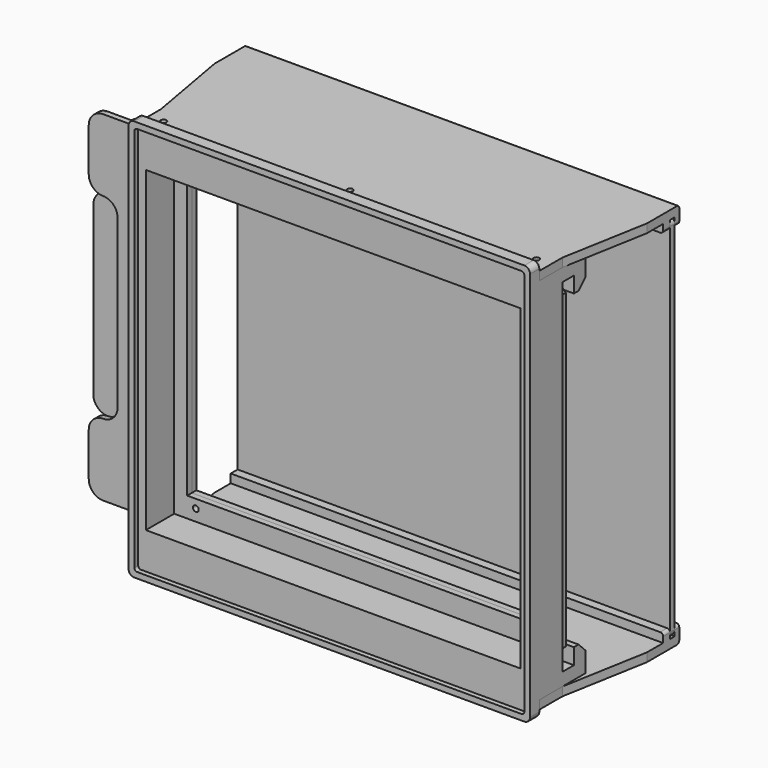
from build123d import *

# Parameters (mm, degrees)
F0_W      = 139.3
F0_H      = 139.3
F0_W_2    = 130
F0_H_2    = 110
F1_DEPTH  = 2.3
F2_W      = 139.3
F2_H      = 128
F2_W_2    = 130
F2_H_2    = 110
F3_DEPTH  = 10
F4_W      = 139.3
F4_H      = 139.3
F4_W_2    = 135.3
F4_H_2    = 135.3
F5_DEPTH  = 1.7
F6_R      = 1
F7_R      = 2
F8_W      = 162.3
F8_H      = 118
F8_W_2    = 121
F8_H_2    = 96
F9_DEPTH  = 2
F10_R     = 1
F11_DEPTH = 25
F12_SIZE  = 5
F13_R     = 1
F13_W     = 121
F13_H     = 96
F14_DEPTH = 2
F15_W     = 10
F15_H     = 25
F16_DEPTH = 25
F17_R     = 4.99999
F18_W     = 10
F18_H     = 68
F19_DEPTH = 25
F20_R     = 4.99999
F21_W     = 139.3
F21_H     = 4.5
F22_DEPTH = 5
F23_W     = 139.3
F23_H     = 10
F24_DEPTH = 5
F25_SIZE  = 3
F27_DEPTH = 75
F28_W     = 2
F28_H     = 128
F29_DEPTH = 150
F30_R     = 2
F31_R     = 1
F31_2_R   = 1
F33_DEPTH = 80
F34_R     = 1
F35_DEPTH = 8
F36_R     = 1
F37_DEPTH = 8


# Not quite as in the source:
# - a fillet or chamfer is up to 0.001 mm smaller than in the source, because OpenCascade refuses the exact size


with BuildPart() as f1:
    # F0 (on Front) → F1 (new body)
    with BuildSketch(Plane.XZ):
        Rectangle(F0_W, F0_H)
        Rectangle(F0_W_2, F0_H_2, mode=Mode.SUBTRACT)
    extrude(amount=F1_DEPTH)

    # F2 (on face) → F3 (join)
    with BuildSketch(Plane(origin=(0, 0, 0), x_dir=(-1, 0, 0), z_dir=(0, 1, 0))):
        Rectangle(F2_W, F2_H)
        Rectangle(F2_W_2, F2_H_2, mode=Mode.SUBTRACT)
    extrude(amount=F3_DEPTH)

    # F4 (on face) → F5 (join)
    with BuildSketch(Plane.XZ.offset(2.3)):
        Rectangle(F4_W, F4_H)
        Rectangle(F4_W_2, F4_H_2, mode=Mode.SUBTRACT)
    extrude(amount=F5_DEPTH)

    # F6
    f6_edges = [f1.edges().sort_by_distance(p)[0] for p in [
        (-67.65, -3.15, 67.65),
        (67.65, -3.15, 67.65),
        (-67.65, -3.15, -67.65),
        (67.65, -3.15, -67.65),
    ]]
    fillet(f6_edges, radius=F6_R)

    # F7
    f7_edges = [f1.edges().sort_by_distance(p)[0] for p in [
        (-69.65, -2, -69.65),
        (69.65, -2, -69.65),
        (69.65, -2, 69.65),
        (-69.65, -2, 69.65),
    ]]
    fillet(f7_edges, radius=F7_R)

    # F21 (on face) → F22 (join)
    with BuildSketch(Plane(origin=(0, 10, 0), x_dir=(-1, 0, 0), z_dir=(0, 1, 0))):
        with Locations((0, 61.75)):
            Rectangle(F21_W, F21_H)
        with Locations((0, -61.75)):
            Rectangle(F21_W, F21_H)
    extrude(amount=F22_DEPTH)

    # F23 (on face) → F24 (join)
    with BuildSketch(Plane(origin=(0, 15, 0), x_dir=(-1, 0, 0), z_dir=(0, 1, 0))):
        with Locations((0, 59)):
            Rectangle(F23_W, F23_H)
        with Locations((0, -59)):
            Rectangle(F23_W, F23_H)
    extrude(amount=F24_DEPTH)

    # F25
    f25_edges = [f1.edges().sort_by_distance(p)[0] for p in [
        (0, 20, 54),
        (0, 20, -54),
    ]]
    chamfer(f25_edges, length=F25_SIZE)


with BuildPart() as f9:
    # F8 (on face) → F9 (new body)
    with BuildSketch(Plane(origin=(0, 10, 0), x_dir=(-1, 0, 0), z_dir=(0, 1, 0))):
        with Locations((13.5, 0)):
            Rectangle(F8_W, F8_H)
        Rectangle(F8_W_2, F8_H_2, mode=Mode.SUBTRACT)
    extrude(amount=F9_DEPTH)

    # F10 (on face) → F11 (cut)
    with BuildSketch(Plane(origin=(0, 12, 0), x_dir=(-1, 0, 0), z_dir=(0, 1, 0))):
        with Locations((-57.5, 51)):
            Circle(F10_R)
        with Locations((57.5, 51)):
            Circle(F10_R)
        with Locations((57.5, -51)):
            Circle(F10_R)
        with Locations((-57.5, -51)):
            Circle(F10_R)
        with Locations((-63.5, 0)):
            Circle(F10_R)
    extrude(amount=-F11_DEPTH, mode=Mode.SUBTRACT)

    # F12
    f12_edges = [f9.edges().sort_by_distance(p)[0] for p in [
        (67.65, 11, -59),
        (67.65, 11, 59),
    ]]
    chamfer(f12_edges, length=F12_SIZE)

    # F18 (on face) → F19 (cut)
    with BuildSketch(Plane(origin=(0, 12, 0), x_dir=(-1, 0, 0), z_dir=(0, 1, 0))):
        with Locations((89.65, 0)):
            Rectangle(F18_W, F18_H)
    extrude(amount=-F19_DEPTH, mode=Mode.SUBTRACT)

    # F20 (radius 5 in the source; OpenCascade refuses exactly that, so slightly less here)
    f20_edges = [f9.edges().sort_by_distance(p)[0] for p in [
        (-94.65, 11, -59),
        (-94.65, 11, -34),
        (-84.65, 11, -34),
        (-84.65, 11, 34),
        (-94.65, 11, 34),
        (-94.65, 11, 59),
    ]]
    fillet(f20_edges, radius=F20_R)


with BuildPart() as f14:
    # F13 (on face) → F14 (new body)
    with BuildSketch(Plane(origin=(0, 12, 0), x_dir=(-1, 0, 0), z_dir=(0, 1, 0))):
        Polygon((94.65, -59), (94.65, 59), (-62.65, 59), (-67.65, 54), (-67.65, -54), (-62.65, -59), align=None)
        with Locations((-57.5, -51)):
            Circle(F13_R, mode=Mode.SUBTRACT)
        with Locations((57.5, -51)):
            Circle(F13_R, mode=Mode.SUBTRACT)
        with Locations((-63.5, 0)):
            Circle(F13_R, mode=Mode.SUBTRACT)
        Rectangle(F13_W, F13_H, mode=Mode.SUBTRACT)
        with Locations((-57.5, 51)):
            Circle(F13_R, mode=Mode.SUBTRACT)
        with Locations((57.5, 51)):
            Circle(F13_R, mode=Mode.SUBTRACT)
    extrude(amount=F14_DEPTH)

    # F15 (on face) → F16 (cut)
    with BuildSketch(Plane(origin=(0, 14, 0), x_dir=(-1, 0, 0), z_dir=(0, 1, 0))):
        with Locations((89.65, 46.5)):
            Rectangle(F15_W, F15_H)
        with Locations((89.65, -46.5)):
            Rectangle(F15_W, F15_H)
    extrude(amount=-F16_DEPTH, mode=Mode.SUBTRACT)

    # F17 (radius 5 in the source; OpenCascade refuses exactly that, so slightly less here)
    f17_edges = [f14.edges().sort_by_distance(p)[0] for p in [
        (-84.65, 13, -59),
        (-84.65, 13, -34),
        (-94.65, 13, -34),
        (-94.65, 13, 34),
        (-84.65, 13, 34),
        (-84.65, 13, 59),
    ]]
    fillet(f17_edges, radius=F17_R)


with BuildPart() as f27:
    # F26 (on Right) → F27 (new body, symmetric)
    with BuildSketch(Plane.YZ):
        Polygon((0, 67), (0, 64), (47, 64), (47, 61), (50, 61), (50, 64), (52, 64), (52, 61), (54, 61), (54, 67), align=None)
    extrude(amount=F27_DEPTH, both=True)

    # F31
    f31_edges = [f27.edges().sort_by_distance(p)[0] for p in [
        (0, 54, 67),
        (75, 53, 61),
        (75, 48.5, 61),
    ]]
    fillet(f31_edges, radius=F31_R)


with BuildPart() as f27b:
    # F26 (on Right) → F27, piece 2 (new body, symmetric)
    with BuildSketch(Plane.YZ):
        Polygon((0, -64), (0, -67), (54, -67), (54, -61), (52, -61), (52, -64), (50, -64), (50, -61), (47, -61), (47, -64), align=None)
    extrude(amount=F27_DEPTH, both=True)

    # F31#2
    f31_2_edges = [f27b.edges().sort_by_distance(p)[0] for p in [
        (0, 54, -67),
        (75, 53, -61),
        (75, 48.5, -61),
    ]]
    fillet(f31_2_edges, radius=F31_2_R)


with BuildPart() as f29:
    # F28 (on face) → F29 (new body, through all)
    with BuildSketch(Plane.YZ.offset(75)):
        with Locations((51, 0)):
            Rectangle(F28_W, F28_H)
    extrude(amount=-F29_DEPTH)

    # F30
    f30_edges = [f29.edges().sort_by_distance(p)[0] for p in [
        (75, 51, 64),
        (75, 51, -64),
    ]]
    fillet(f30_edges, radius=F30_R)


with BuildPart() as f33_tool:
    # F32 (on Top) → F33 (new body, symmetric)
    with BuildSketch(Plane.XY):
        Polygon((-75, 0), (-69.65, 0), (-69.65, 10), (-75, 40), align=None)
        Polygon((75, 0), (75, 40), (69.65, 10), (69.65, 0), align=None)
    extrude(amount=F33_DEPTH, both=True)


with BuildPart() as f27_1:
    add(f27.part)

    # F33: cut by f33_tool
    add(f33_tool.part, mode=Mode.SUBTRACT)


with BuildPart() as f27b_1:
    add(f27b.part)

    # F33: cut by f33_tool
    add(f33_tool.part, mode=Mode.SUBTRACT)


with BuildPart() as f35_tool:
    # F34 (on face) → F35 (new body)
    with BuildSketch(Plane(origin=(0, 0, -67), x_dir=(1, 0, 0), z_dir=(0, 0, -1))):
        with Locations((-64.65, -5)):
            Circle(F34_R)
        with Locations((0, -5)):
            Circle(F34_R)
        with Locations((64.65, -5)):
            Circle(F34_R)
    extrude(amount=-F35_DEPTH)


with BuildPart() as f1_1:
    add(f1.part)

    # F35: cut by f35_tool
    add(f35_tool.part, mode=Mode.SUBTRACT)


with BuildPart() as f27b_2:
    add(f27b_1.part)

    # F35: cut by f35_tool
    add(f35_tool.part, mode=Mode.SUBTRACT)


with BuildPart() as f37_tool:
    # F36 (on face) → F37 (new body)
    with BuildSketch(Plane.XY.offset(67)):
        with Locations((-64.65, 5)):
            Circle(F36_R)
        with Locations((0, 5)):
            Circle(F36_R)
        with Locations((64.65, 5)):
            Circle(F36_R)
    extrude(amount=-F37_DEPTH)


with BuildPart() as f1_2:
    add(f1_1.part)

    # F37: cut by f37_tool
    add(f37_tool.part, mode=Mode.SUBTRACT)


with BuildPart() as f27_2:
    add(f27_1.part)

    # F37: cut by f37_tool
    add(f37_tool.part, mode=Mode.SUBTRACT)


solid = Compound([f9.part, f14.part, f29.part, f27b_2.part, f1_2.part, f27_2.part])
